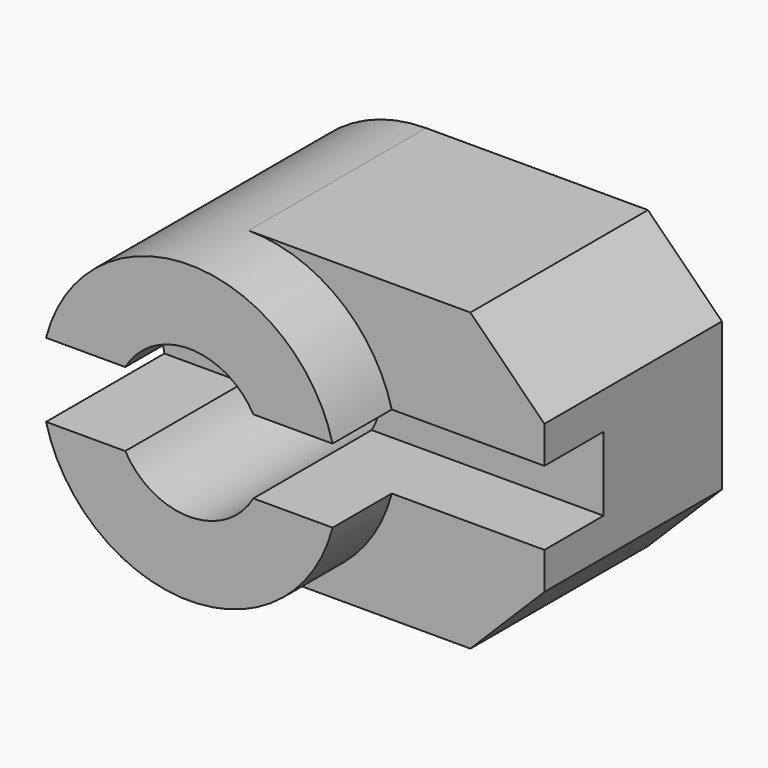
from build123d import *
from build123d import SkipClean  # not in build123d's __all__

# Parameters (mm, degrees)
F0_R     = 10
F0_R_2   = 5
F1_DEPTH = 10
F3_DEPTH = 10
F5_DEPTH = 5
F7_DEPTH = 10


with BuildPart() as f1:
    # F0 (on Front) → F1 (new body, symmetric)
    with BuildSketch(Plane.XZ):
        Circle(F0_R)
        Circle(F0_R_2, mode=Mode.SUBTRACT)
    extrude(amount=F1_DEPTH, both=True)

    # F2 (on Front) → F3 (join, symmetric)
    with BuildSketch(Plane.XZ):
        with BuildLine():
            Line((15, 10), (0, 10))
            ThreePointArc((0, 10), (10, 0), (0, -10))
            Line((0, -10), (15, -10))
            Line((15, -10), (20, -5))
            Line((20, -5), (20, 5))
            Line((20, 5), (15, 10))
        make_face()
    extrude(amount=F3_DEPTH, both=True)

    # F4 (on face) → F5 (cut)
    with BuildSketch(Plane.XZ.offset(10)):
        with BuildLine():
            ThreePointArc((0, 10), (10, 0), (0, -10))
            Line((0, -10), (15, -10))
            Line((15, -10), (20, -5))
            Line((20, -5), (20, 5))
            Line((20, 5), (15, 10))
            Line((15, 10), (0, 10))
        make_face()
    with SkipClean():  # cleaning this boolean's faces spoils the solid; the shape is the same uncleaned
        extrude(amount=-F5_DEPTH, mode=Mode.SUBTRACT)

    # F6 (on Front) → F7 (cut)
    with BuildSketch(Plane.XZ):
        with BuildLine():
            Line((20.3175416345, 2.5), (-9.6824583655, 2.5))
            ThreePointArc((-9.6824583655, 2.5), (-10, 0), (-9.6824583655, -2.5))
            Line((-9.6824583655, -2.5), (20.3175416345, -2.5))
            Line((20.3175416345, -2.5), (20.3175416345, 2.5))
        make_face()
    extrude(amount=F7_DEPTH, mode=Mode.SUBTRACT)


solid = f1.part
